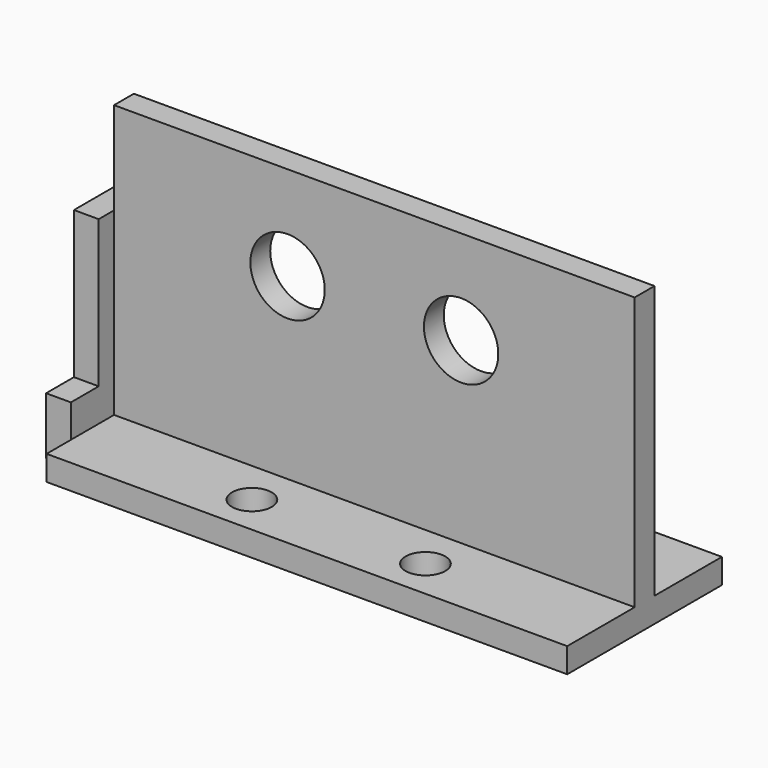
from build123d import *

# Parameters (mm, degrees)
F1_DEPTH     = 52.5
F3_D         = 8
F6_D         = 15
F8_DEPTH     = 5
F9_T         = -2.5
F10_T        = 2.5
F10_T3_DEPTH = 110


# Not quite as in the source:
# - a shell that OpenCascade refuses in one call is made with other operations: the cavity is built on its own and cut out


with BuildPart() as f1:
    # F0 (on Right) → F1 (new body, symmetric)
    with BuildSketch(Plane.YZ):
        Polygon((-13.3118266579, 0), (-13.3118266579, 55), (-18.3118266579, 55), (-18.3118266579, 0), (-35.3118266579, 0), (-35.3118266579, -5), (-13.3118266579, -5), (3.6881733421, -5), (3.6881733421, 0), align=None)
    extrude(amount=F1_DEPTH, both=True)

    # F3 (through all)
    with Locations(Plane(origin=(0, 0, -5), x_dir=(1, 0, 0), z_dir=(0, 0, -1))):
        with Locations((-17.5, 27.3118266579), (17.5, 27.3118266579), (-17.5, 4.3118266579), (17.5, 4.3118266579)):
            Hole(F3_D / 2)

    # F6 (through all)
    with Locations(Plane.XZ.offset(18.3118266579)):
        with Locations((17.5, 36), (-17.5, 36)):
            Hole(F6_D / 2)

    # F10: shell of thickness 2.5, made by hand


with BuildPart() as f8:
    # F7 (on offset) → F8 (new body)
    with BuildSketch(Plane(origin=(-52.5, 0, 0), x_dir=(0, -1, 0), z_dir=(-1, 0, 0))):
        Polygon((2.3793176152, 6.649301853), (2.3793176152, -4.9209868232), (29.1948146988, -4.9209868232), (29.1948146988, 6.649301853), (22.175675258, 6.649301853), (22.175675258, 36.3233052194), (8.4276301786, 36.3233052194), (8.4276301786, 6.649301853), align=None)
    extrude(amount=F8_DEPTH)

    # F9
    f9_openings = [f8.faces().sort_by_distance(p)[0] for p in [
        (-57.5, -15.511345, 12.577798),
    ]]
    offset(amount=F9_T, openings=f9_openings, kind=Kind.INTERSECTION)


with BuildPart() as f10_core1:
    # F10_t2: copy of F1
    add(f1.part)

    # the walls: a layer under each face that stays
    f10_faces = [f10_core1.faces().sort_by_distance(p)[0] for p in [
        (0, -4.8118266579, 0),
        (-52.5, -15.8118266579, 25),
        (0, 3.6881733421, -2.5),
        (0, -13.3118266579, 27.5),
        (52.5, -15.8118266579, 25),
        (-21.5, -4.3118266579, -2.5),
        (13.5, -4.3118266579, -2.5),
        (0, -15.8118266579, 55),
        (0, -18.3118266579, 27.5),
        (0, -26.8118266579, 0),
        (0, -35.3118266579, -2.5),
        (-25, -15.8118266579, 36),
        (10, -15.8118266579, 36),
        (-21.5, -27.3118266579, -2.5),
        (13.5, -27.3118266579, -2.5),
    ]]
    thicken(f10_faces, amount=-F10_T, mode=Mode.SUBTRACT)

    # F10_s4 → F10_t3 (cut)
    with BuildSketch(Plane.YZ.offset(-55)):
        Polygon((-13.2868266579, 0.025), (-13.3118266579, -2.5), (-15.8118266579, -2.5), (-15.8118266579, 0), align=None)
        Polygon((-18.3368266579, 0.025), (-15.8118266579, 0), (-15.8118266579, -2.5), (-18.3118266579, -2.5), align=None)
    extrude(amount=F10_T3_DEPTH, mode=Mode.SUBTRACT)


with BuildPart() as f1_1:
    add(f1.part)

    # what is left inside the walls is the cavity
    f10_cavity = [f10_core1.part.solids().sort_by_distance(p)[0] for p in [
        (-16.666667, -15.811827, -4.975),
    ]]
    add(f10_cavity, mode=Mode.SUBTRACT)


solid = Compound([f8.part, f1_1.part])
